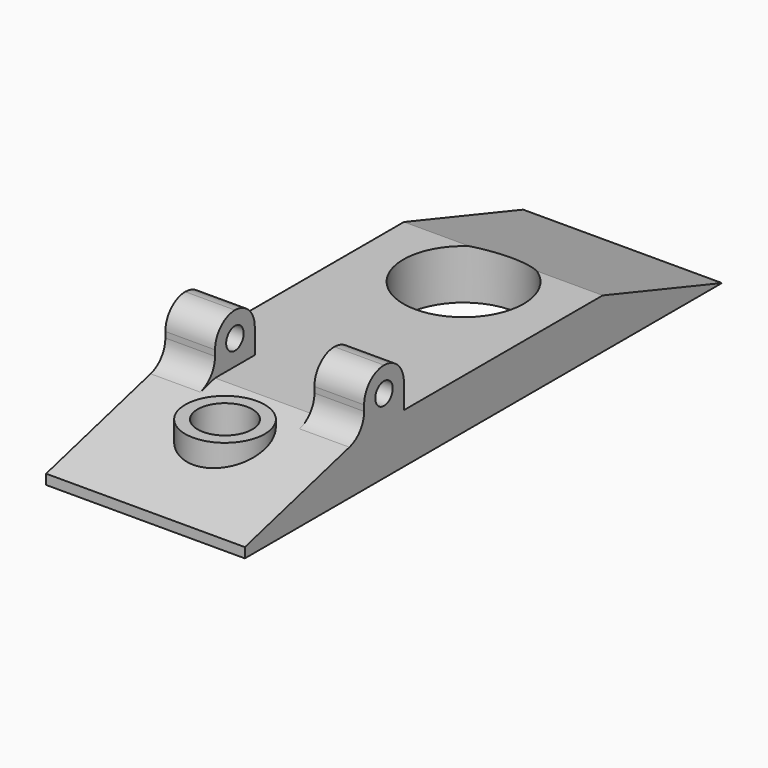
from build123d import *

# Parameters (mm, degrees)
F0_W         = 20
F0_H         = 60
F0_R         = 4
F0_R_2       = 6.05
F1_DEPTH     = 4
F1_FACE_W    = 20
F1_FACE_H    = 60
F1_FACE_R    = 4
F1_FACE_R_2  = 6.05
F0_R_3       = 2.75
F2_DEPTH     = 1
F3_W         = 5
F3_H         = 5
F4_DEPTH     = 5
F5_T1_DEPTH  = 97.9025398997
F6_R         = 2.49999
F7_R         = 1.1
F8_DEPTH     = 25
F9_DEPTH     = 5
F10_T1_DEPTH = 97.8518303197
F11_DEPTH    = 2


# Not quite as in the source:
# - a fillet or chamfer that OpenCascade refuses, or shapes differently, is made with other operations: its cross-section is extruded or revolved along the edge and cut away or added
# - a fillet or chamfer is up to 0.001 mm smaller than in the source, because OpenCascade refuses the exact size


with BuildPart() as f1:
    # F0 (on Top) → F1 (new body)
    with BuildSketch(Plane.XY):
        with Locations((10, 30)):
            Rectangle(F0_W, F0_H)
        with Locations((10, 10)):
            Circle(F0_R, mode=Mode.SUBTRACT)
        with Locations((10, 40)):
            Circle(F0_R_2, mode=Mode.SUBTRACT)
    extrude(amount=F1_DEPTH)

    # F1_face (on face) + F0 (on Top) → F2 (join)
    with BuildSketch(Plane(origin=(10, 29.8602632633, 4), x_dir=(1, 0, 0), z_dir=(0, 0, 1))):
        with Locations((0, 0.1397367367)):
            Rectangle(F1_FACE_W, F1_FACE_H)
        with Locations((0, -19.8602632633)):
            Circle(F1_FACE_R, mode=Mode.SUBTRACT)
        with Locations((0, 10.1397367367)):
            Circle(F1_FACE_R_2, mode=Mode.SUBTRACT)
    with BuildSketch(Plane.XY):
        with Locations((10, 10)):
            Circle(F0_R)
        with Locations((10, 10)):
            Circle(F0_R_3, mode=Mode.SUBTRACT)
    extrude(amount=F2_DEPTH)

    # F3 (on face) → F4 (join)
    with BuildSketch(Plane.XY.offset(5)):
        with Locations((2.5, 17.5)):
            Rectangle(F3_W, F3_H)
        with Locations((17.5, 17.5)):
            Rectangle(F3_W, F3_H)
    extrude(amount=F4_DEPTH)

    # F5: chamfer of 15 x 4 on 1 edges, made by hand

    # F5_s2 → F5_t1 (cut)
    with BuildSketch(Plane.YZ.offset(-38.9512699498)):
        Polygon((15, 5), (0, 1), (0, 5), align=None)
    extrude(amount=F5_T1_DEPTH, mode=Mode.SUBTRACT)

    # F6 (radius 2.5 in the source; OpenCascade refuses exactly that, so slightly less here)
    f6_edges = [f1.edges().sort_by_distance(p)[0] for p in [
        (2.5, 15, 5),
        (2.5, 15, 10),
        (17.5, 15, 5),
        (17.5, 15, 10),
        (2.5, 20, 10),
        (17.5, 20, 10),
    ]]
    fillet(f6_edges, radius=F6_R)

    # F7 (on face) → F8 (cut)
    with BuildSketch(Plane(origin=(0, 0, 0), x_dir=(0, -1, 0), z_dir=(-1, 0, 0))):
        with Locations((-17.5, 7.5)):
            Circle(F7_R)
    extrude(amount=-F8_DEPTH, mode=Mode.SUBTRACT)

    # F10: chamfer of 5 x 15 on 1 edges, made by hand

    # F10_s2 → F10_t1 (cut)
    with BuildSketch(Plane.YZ.offset(-38.9259151598)):
        Polygon((60, 0), (45, 5), (60, 5), align=None)
    extrude(amount=F10_T1_DEPTH, mode=Mode.SUBTRACT)



with BuildPart() as f9:
    # F0 (on Top) → F9 (new body)
    with BuildSketch(Plane.XY):
        with Locations((10, 10)):
            Circle(F0_R)
        with Locations((10, 10)):
            Circle(F0_R_3, mode=Mode.SUBTRACT)
    extrude(amount=F9_DEPTH)


with BuildPart() as f1_1:
    add(f1.part)

    add(f9.part)  # F11 merges F9
    # F0 (on Top) → F11 (join)
    with BuildSketch(Plane.XY):
        with Locations((10, 10)):
            Circle(F0_R_3)
    extrude(amount=F11_DEPTH)


solid = f1_1.part
